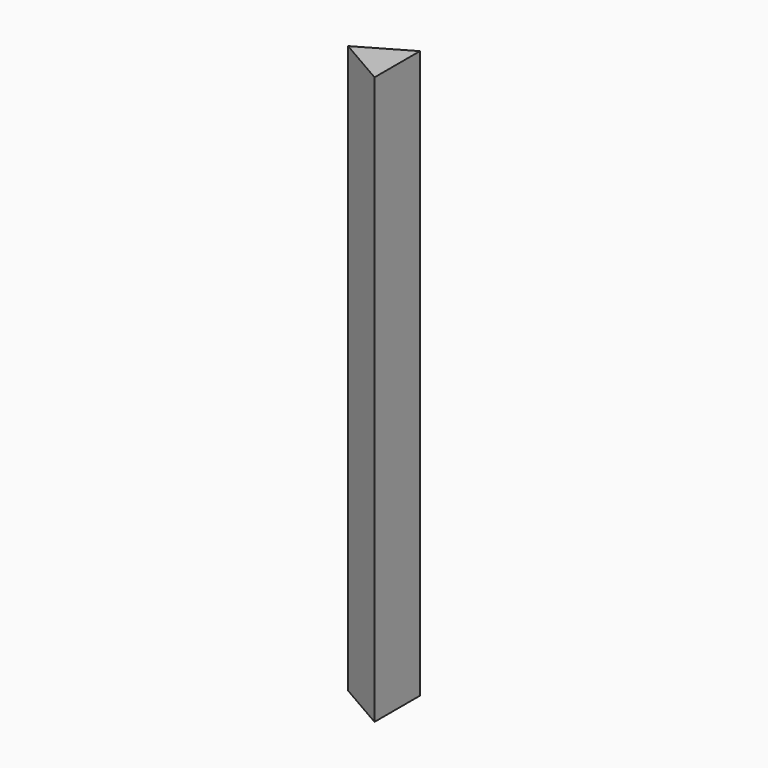
from build123d import *

# Parameters (mm, degrees)
F1_DEPTH = 25.4


# Not quite as in the source:
# - the program builds the solid bodies; features that only make, move or delete a surface that nothing else refers to are left out


with BuildPart() as f1:
    # F0 (on Top) → F1 (new body)
    with BuildSketch(Plane.XY):
        Polygon((-36.3498746287, -35.8157656759), (-38.5495791543, -37.0857656759), (-36.3498746287, -38.3557656759), align=None)
    extrude(amount=F1_DEPTH)


solid = f1.part
